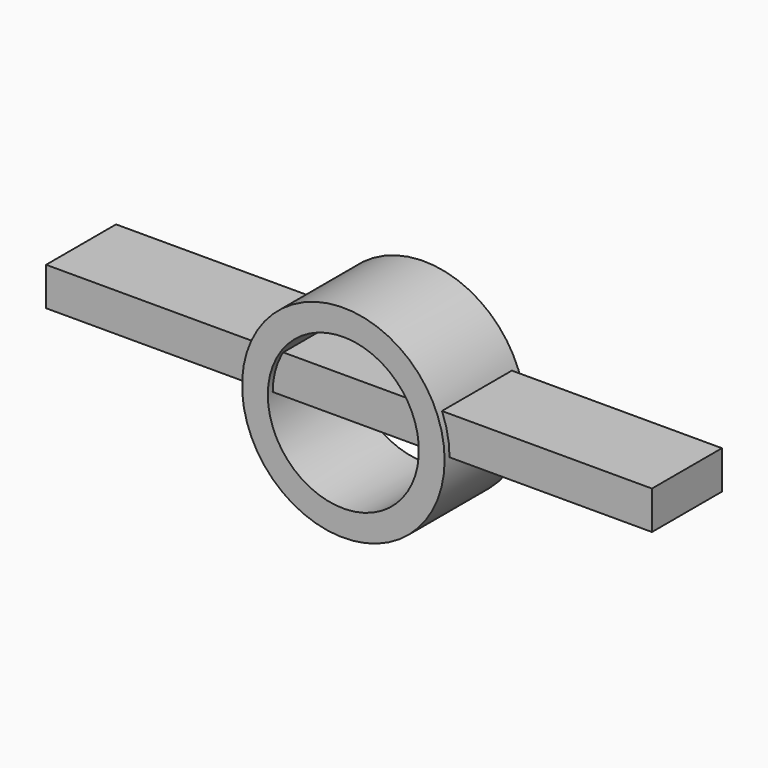
from build123d import *

# Parameters (mm, degrees)
F0_R          = 25.5397
F1_DEPTH      = 25.4
F3_D          = 38.1
F4_W          = 22.0553190447
F4_H          = 9.6537293866
F5_DEPTH      = 25.5407
F5_DEPTH_BACK = 76.2


# Not quite as in the source:
# - a pattern or mirror of a feature is missing from the dataset's text; its kind, count and spacing are read off the source's solid


with BuildPart() as f1:
    # F0 (on Front) → F1 (new body)
    with BuildSketch(Plane.XZ):
        Circle(F0_R)
    extrude(amount=F1_DEPTH)

    # F3 (through all)
    with Locations(Plane.XZ.offset(25.4)):
        with Locations((0, 0)):
            Hole(F3_D / 2)


with BuildPart() as f5:
    # F4 (on Right) → F5 (new body, two sides)
    with BuildSketch(Plane.YZ) as f5_sk:
        with Locations((-12.8223716747, 4.8268646933)):
            Rectangle(F4_W, F4_H)
    extrude(amount=F5_DEPTH)
    extrude(f5_sk.sketch, amount=-F5_DEPTH_BACK)

    # F5_copies: F5 across plane


with BuildPart() as f5_1:
    add(f5.part)
    add(f5.part.mirror(Plane(origin=(0.191323, 0, 0), x_dir=(0, 0, 1), z_dir=(1, 0, 0))))


solid = Compound([f1.part, f5_1.part])
